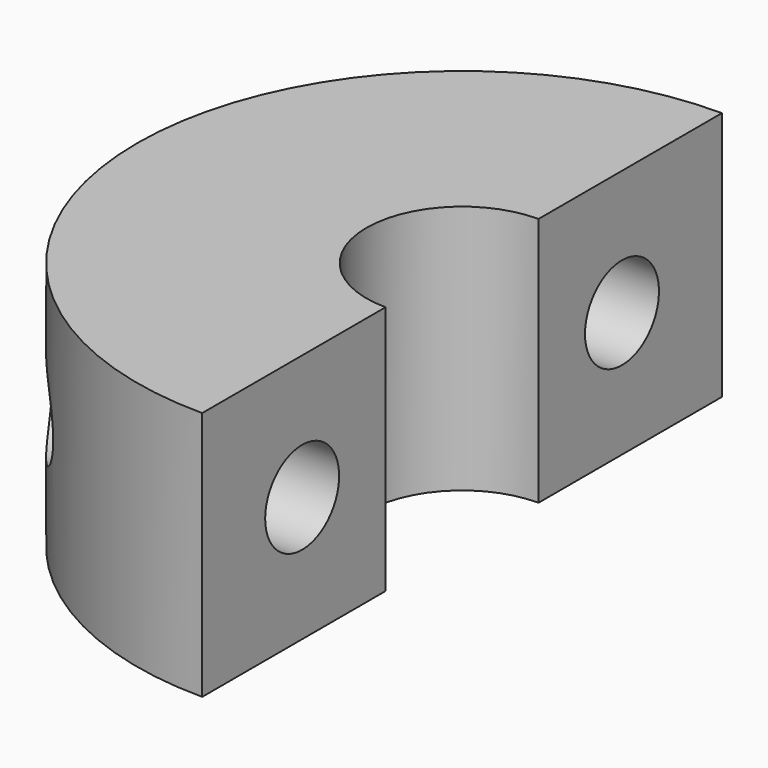
from build123d import *

# Parameters (mm, degrees)
F0_W        = 6.7956063077
F0_H        = 13
F0_H_2      = 6.5
F0_W_2      = 6.2043936923
F1_DEPTH    = 10
F2_R        = 1.85
F3_DEPTH    = 13
F4_T1_DEPTH = 75


# Not quite as in the source:
# - a fillet or chamfer that OpenCascade refuses, or shapes differently, is made with other operations: its cross-section is extruded or revolved along the edge and cut away or added
# - a feature names something its author has since deleted; it is built from what else it names


with BuildPart() as f1:
    # F0 (on Top) → F1 (new body)
    with BuildSketch(Plane.XY):
        with BuildLine():
            Line((0, 6.5), (-6.2043936923, 6.5))
            Line((-6.2043936923, 6.5), (-6.2043936923, -6.5))
            Line((-6.2043936923, -6.5), (0, -6.5))
            Line((0, -6.5), (0, -3.825))
            ThreePointArc((0, -3.825), (-3.825, 0), (0, 3.825))
            Line((0, 3.825), (0, 6.5))
        make_face()
        with Locations((-9.6021968462, 0)):
            Rectangle(F0_W, F0_H)
        with Locations((-9.6021968462, 9.75)):
            Rectangle(F0_W, F0_H_2)
        with Locations((-3.1021968462, 9.75)):
            Rectangle(F0_W_2, F0_H_2)
        Polygon((-6.2043936923, -6.5), (-13, -6.5), (-13, -13), (0, -13), (0, -6.5), align=None)
    extrude(amount=-F1_DEPTH)

    # F2 (on face) → F3 (cut, through all)
    with BuildSketch(Plane(origin=(-13, 0, 0), x_dir=(0, -1, 0), z_dir=(-1, 0, 0))):
        with Locations((-8, -5)):
            Circle(F2_R)
        with Locations((8, -5)):
            Circle(F2_R)
    extrude(amount=-F3_DEPTH, mode=Mode.SUBTRACT)

    # F4: fillet of radius 13 on 2 edges, made by hand

    # F4_s2 → F4_t1 (cut)
    with BuildSketch(Plane.XY.offset(-42.5)):
        with BuildLine():
            ThreePointArc((0, 13), (-9.1923881554, 9.1923881554), (-13, 0))
            Line((-13, 0), (-13, 13))
            Line((-13, 13), (0, 13))
        make_face()
        with BuildLine():
            ThreePointArc((0, -13), (-9.1923881554, -9.1923881554), (-13, 0))
            Line((-13, 0), (-13, -13))
            Line((-13, -13), (0, -13))
        make_face()
    extrude(amount=F4_T1_DEPTH, mode=Mode.SUBTRACT)


solid = f1.part
